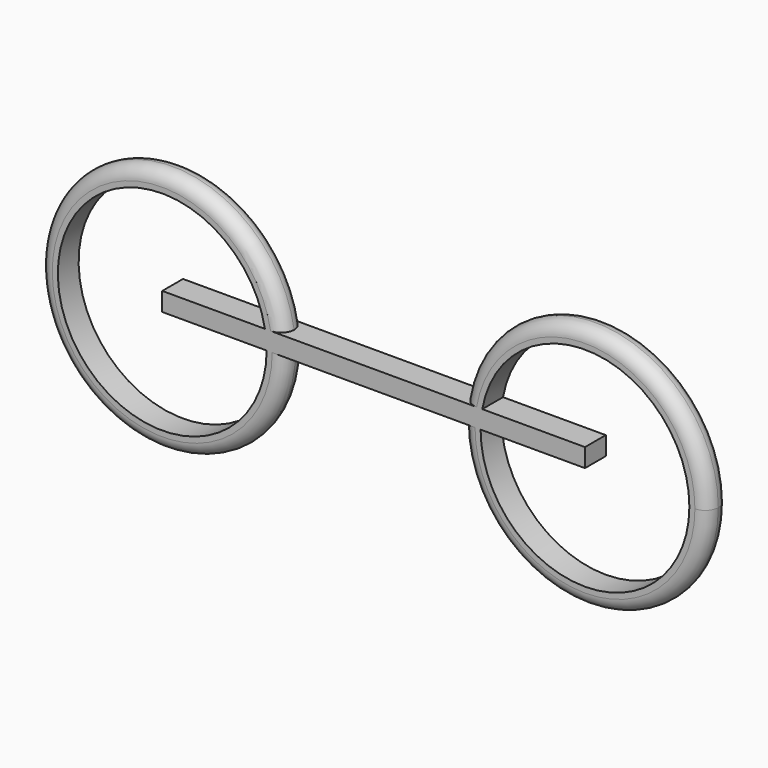
from build123d import *

# Parameters (mm, degrees)
F0_R     = 331.5
F0_R_2   = 281.5
F1_DEPTH = 70
F2_R     = 34.99999
F4_W     = 1140
F4_H     = 50
F5_DEPTH = 70


# Not quite as in the source:
# - a fillet or chamfer is up to 0.001 mm smaller than in the source, because OpenCascade refuses the exact size


with BuildPart() as f1:
    # F0 (on Front) → F1 (new body)
    with BuildSketch(Plane.XZ):
        Circle(F0_R)
        Circle(F0_R_2, mode=Mode.SUBTRACT)
    extrude(amount=F1_DEPTH)

    # F2 (radius 35 in the source; OpenCascade refuses exactly that, so slightly less here)
    f2_edges = [f1.edges().sort_by_distance(p)[0] for p in [
        (-331.5, -70, 0),
        (-331.5, 0, 0),
    ]]
    fillet(f2_edges, radius=F2_R)


with BuildPart() as f3_1:
    # F3: copy of F1
    add(f1.part.moved(Location((1140, 0, 0))))


with BuildPart() as f1_1:
    add(f1.part)

    add(f3_1.part)  # F5 merges F3_1
    # F4 (on Front) → F5 (join)
    with BuildSketch(Plane.XZ):
        with Locations((570, 25)):
            Rectangle(F4_W, F4_H)
    extrude(amount=F5_DEPTH)


solid = f1_1.part
